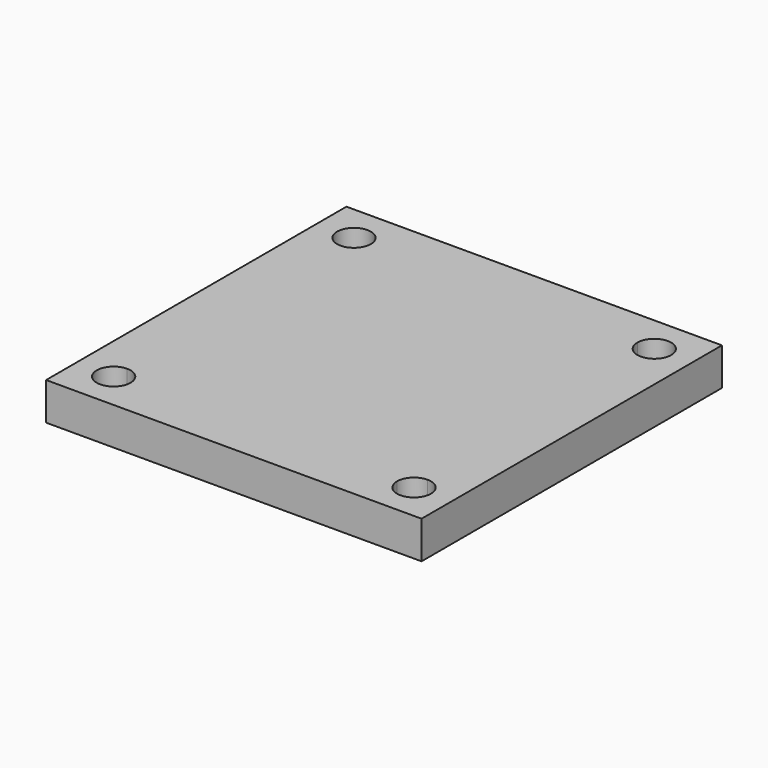
from build123d import *

# Parameters (mm, degrees)
F0_W     = 127
F0_H     = 127
F2_DEPTH = 12.7


# Not quite as in the source:
# - the program builds the solid bodies; features that only make, move or delete a surface that nothing else refers to are left out


with BuildPart() as f2:
    # F0 (on Top) → F2 (new body)
    with BuildSketch(Plane.XY):
        Rectangle(F0_W, F0_H)
        with BuildLine():
            ThreePointArc((-50.8, 45.085), (-54.8411152545, 54.8411152545), (-45.085, 50.8))
            Line((-45.085, 50.8), (45.085, 50.8))
            ThreePointArc((45.085, 50.8), (50.8, 56.515), (56.515, 50.8))
            ThreePointArc((56.515, 50.8), (54.8411152545, 46.7588847455), (50.8, 45.085))
            Line((50.8, 45.085), (50.8, -45.085))
            ThreePointArc((50.8, -45.085), (54.8411152545, -46.7588847455), (56.515, -50.8))
            ThreePointArc((56.515, -50.8), (50.8, -56.515), (45.085, -50.8))
            Line((45.085, -50.8), (-45.085, -50.8))
            ThreePointArc((-45.085, -50.8), (-54.8411152545, -54.8411152545), (-50.8, -45.085))
            Line((-50.8, -45.085), (-50.8, 45.085))
        make_face(mode=Mode.SUBTRACT)
        with BuildLine():
            Line((45.085, 50.8), (-45.085, 50.8))
            ThreePointArc((-45.085, 50.8), (-46.7588847455, 46.7588847455), (-50.8, 45.085))
            Line((-50.8, 45.085), (-50.8, -45.085))
            ThreePointArc((-50.8, -45.085), (-46.7588847455, -46.7588847455), (-45.085, -50.8))
            Line((-45.085, -50.8), (45.085, -50.8))
            ThreePointArc((45.085, -50.8), (46.7588847455, -46.7588847455), (50.8, -45.085))
            Line((50.8, -45.085), (50.8, 45.085))
            ThreePointArc((50.8, 45.085), (46.7588847455, 46.7588847455), (45.085, 50.8))
        make_face()
    extrude(amount=F2_DEPTH)


solid = f2.part
